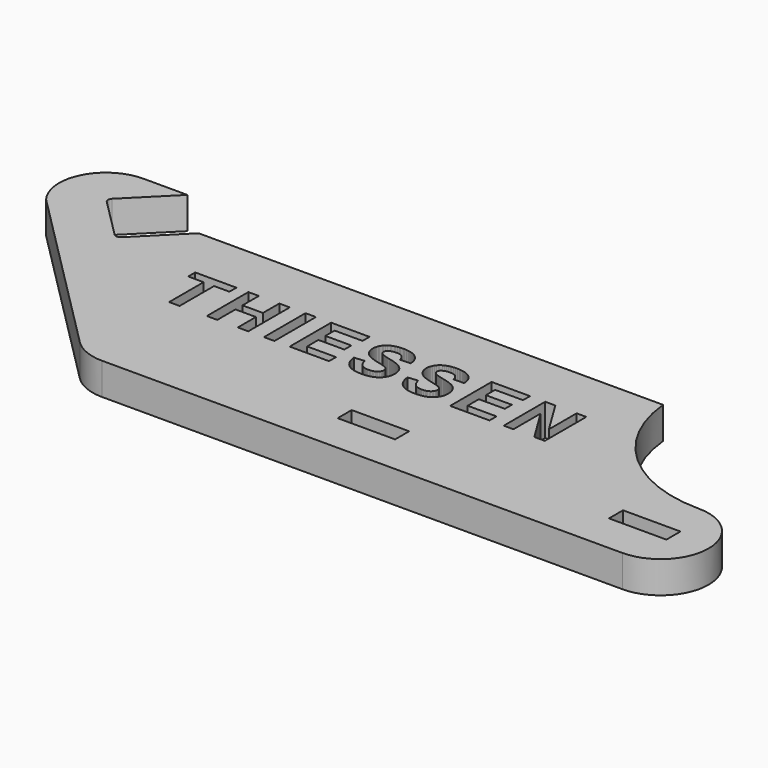
from build123d import *

# Parameters (mm, degrees)
F0_W     = 45.72
F0_H     = 13.97
F0_W_2   = 8.33755
F0_H_2   = 41.275
F1_DEPTH = 25.4


# Not quite as in the source:
# - ends of sketch curves that miss each other by under 0.0002 mm in the source are joined


with BuildPart() as f1:
    # F0 (on Top) → F1 (new body)
    with BuildSketch(Plane.XY):
        with BuildLine():
            Line((-272.2032402, 70.4585586), (-238.976281, 103.6855178))
            Line((-238.976281, 103.6855178), (-273.9992996, 103.6855178))
            ThreePointArc((-273.9992996, 103.6855178), (-307.3025453403, 83.0573981079), (-303.6687029451, 44.0520184737))
            Line((-303.6687029451, 44.0520184737), (-167.3257004, -92.790645))
            ThreePointArc((-167.3257004, -92.790645), (-155.2579794367, -100.8540315519), (-141.0231368, -103.6855178))
            Line((-141.0231368, -103.6855178), (273.096736, -103.6855178))
            ThreePointArc((273.096736, -103.6855178), (311.196736, -65.5855178), (273.096736, -27.4855178))
            ThreePointArc((273.096736, -27.4855178), (202.2970835909, -0.11388545), (168.321736, 67.7644822))
            Line((168.321736, 67.7644822), (-201.2592114, 67.7644822))
            Line((-201.2592114, 67.7644822), (-235.3841876, 33.639506))
            ThreePointArc((-235.3841876, 33.639506), (-238.078264, 32.5235824), (-240.7723408363, 33.6395055637))
            Line((-240.7723408363, 33.6395055637), (-272.2032402, 65.0704058))
            ThreePointArc((-272.2032402, 65.0704058), (-273.3191638, 67.7644822), (-272.2032402, 70.4585586))
        make_face()
        with Locations((44.496736, -65.5855178)):
            Rectangle(F0_W, F0_H, mode=Mode.SUBTRACT)
        with Locations((260.396736, -65.5855178)):
            Rectangle(F0_W, F0_H, mode=Mode.SUBTRACT)
        Polygon((-149.3758506, -16.014827), (-157.7134006, -16.014827), (-157.7134006, 18.284698), (-169.9720756, 18.284698), (-169.9720756, 25.260173), (-137.1584506, 25.260173), (-137.1584506, 18.284698), (-149.3758506, 18.284698), align=None, mode=Mode.SUBTRACT)
        Polygon((-119.3595276, -16.014827), (-127.6970776, -16.014827), (-127.6970776, 25.260173), (-119.3595276, 25.260173), (-119.3595276, 8.997823), (-103.0559026, 8.997823), (-103.0559026, 25.260173), (-94.7183526, 25.260173), (-94.7183526, -16.014827), (-103.0559026, -16.014827), (-103.0559026, 2.022348), (-119.3595276, 2.022348), align=None, mode=Mode.SUBTRACT)
        with Locations((-78.075155, 4.622673)):
            Rectangle(F0_W_2, F0_H_2, mode=Mode.SUBTRACT)
        Polygon((-30.4757074, -16.014827), (-61.8034324, -16.014827), (-61.8034324, 25.260173), (-31.2599324, 25.260173), (-31.2599324, 18.284698), (-53.4658824, 18.284698), (-53.4658824, 9.121648), (-32.7871074, 9.121648), (-32.7871074, 2.146173), (-53.4658824, 2.146173), (-53.4658824, -9.039352), (-30.4757074, -9.039352), align=None, mode=Mode.SUBTRACT)
        Polygon((-21.2402166, -3.6873688), (-21.3858094, -2.641727), (-13.2959094, -1.857502), (-13.0892042, -2.8459176), (-12.8354074, -3.7664898), (-12.5344936, -4.6191678), (-12.1864882, -5.4040024), (-11.7913912, -6.1209682), (-11.3491772, -6.7700398), (-10.8598716, -7.351268), (-10.3234744, -7.8646274), (-9.7390966, -8.3140804), (-9.1058492, -8.7036148), (-8.423783, -9.0332052), (-7.6928472, -9.302877), (-6.9130418, -9.5126302), (-6.0843922, -9.6624394), (-5.2068984, -9.75233), (-4.2805604, -9.782302), (-3.3043876, -9.755632), (-2.3902924, -9.6756728), (-1.5382748, -9.5424244), (-0.7483094, -9.355836), (-0.020447, -9.1159584), (0.6453632, -8.8227662), (1.2490958, -8.4762848), (1.7907508, -8.0764888), (2.4148288, -7.4918316), (2.925445, -6.8750688), (3.3225994, -6.2262004), (3.6062666, -5.5452264), (3.776472, -4.8321722), (3.8332156, -4.086987), (3.7377878, -3.158236), (3.4515552, -2.3264876), (2.9744924, -1.5917926), (2.46507, -1.0939018), (1.7955006, -0.6295644), (0.9657842, -0.198755), (-0.0240792, 0.1985264), (-0.448564, 0.337566), (-0.9900412, 0.501269), (-1.6485108, 0.68961), (-2.4239982, 0.9026144), (-3.3164526, 1.1402568), (-4.3258994, 1.4025372), (-5.4523386, 1.689481), (-6.6957956, 2.0010628), (-7.7848206, 2.2833584), (-8.8183212, 2.576195), (-9.7962974, 2.8796234), (-10.7187492, 3.1935928), (-11.5856512, 3.518154), (-12.3970542, 3.8532816), (-13.1529328, 4.1989756), (-13.853287, 4.555236), (-14.4980914, 4.9220882), (-15.0873968, 5.2994814), (-15.6211524, 5.6874664), (-16.0993836, 6.0860178), (-16.7589962, 6.718173), (-17.3557692, 7.375017), (-17.889728, 8.0565498), (-18.3608726, 8.762746), (-18.7691776, 9.493631), (-19.1146938, 10.2491794), (-19.3973704, 11.0294166), (-19.6172328, 11.8343172), (-19.774281, 12.6639066), (-19.868515, 13.5181594), (-19.8999094, 14.3971264), (-19.863435, 15.2903682), (-19.7540372, 16.166973), (-19.5716906, 17.0268646), (-19.3163952, 17.8701192), (-18.988151, 18.6966606), (-18.586958, 19.506565), (-18.1128416, 20.2997562), (-17.641443, 20.966049), (-17.1207938, 21.591397), (-16.5508686, 22.1758002), (-15.9317182, 22.7192586), (-15.2632918, 23.2217976), (-14.5456148, 23.6833664), (-13.7786872, 24.1039904), (-12.9624836, 24.483695), (-12.1978928, 24.7852692), (-11.3989104, 25.0513596), (-10.5655364, 25.2819662), (-9.6977454, 25.477089), (-8.7955882, 25.6367534), (-7.859014, 25.760934), (-6.8880482, 25.8496308), (-5.8826908, 25.9028438), (-4.8429164, 25.920573), (-3.7529008, 25.9031994), (-2.702052, 25.8510278), (-1.6903954, 25.7640582), (-0.7179564, 25.6423414), (0.2152904, 25.4858266), (1.1093704, 25.2945392), (1.9642328, 25.0684792), (2.779903, 24.8076212), (3.5563556, 24.5119906), (4.2936414, 24.1815874), (4.991735, 23.8164116), (5.650611, 23.4164378), (6.2702948, 22.9816914), (6.8507864, 22.5121724), (7.479284, 21.9282518), (8.0559656, 21.3126574), (8.5808312, 20.6653892), (9.0539316, 19.9864472), (9.4751906, 19.275806), (9.8446844, 18.533491), (10.1623622, 17.7594768), (10.4282494, 16.9537888), (10.6423206, 16.116427), (10.8046266, 15.2473914), (10.9150912, 14.3466566), (10.9737906, 13.414248), (2.6362406, 13.042773), (2.424049, 14.0562584), (2.1439124, 14.9701504), (1.7958054, 15.7844998), (1.3797788, 16.4992812), (0.8957818, 17.1144692), (0.3438652, 17.6301146), (-0.1942338, 18.0008784), (-0.8041132, 18.3146192), (-1.4857476, 18.5713116), (-2.239137, 18.7709556), (-3.0643322, 18.9135766), (-3.9612824, 18.9991238), (-4.9299876, 19.027648), (-5.9345068, 18.9971426), (-6.874764, 18.9055756), (-7.7507338, 18.752947), (-8.5623908, 18.5393076), (-9.3098112, 18.2646066), (-9.9929188, 17.9288694), (-10.6117644, 17.5320706), (-11.1901732, 17.0119802), (-11.6033296, 16.4107114), (-11.8512082, 15.7282642), (-11.9338344, 14.9646386), (-11.8564152, 14.2574772), (-11.6241322, 13.603224), (-11.23696, 13.0018282), (-10.6949494, 12.4533152), (-10.3345234, 12.1870216), (-9.8839782, 11.9185182), (-9.3433392, 11.6477796), (-8.7125556, 11.3748566), (-7.9916782, 11.0996984), (-7.1806816, 10.8223558), (-6.2795658, 10.542778), (-5.2883308, 10.2609904), (-4.207002, 9.976993), (-3.0355286, 9.6907858), (-1.9558, 9.4287848), (-0.9284208, 9.1651836), (0.0465836, 8.8999568), (0.9692386, 8.6331044), (1.8394934, 8.3646518), (2.6573988, 8.0945736), (3.4229548, 7.8228698), (4.136136, 7.5495658), (4.7969424, 7.2746616), (5.405374, 6.9981064), (5.9614562, 6.7199764), (6.7682872, 6.2586362), (7.5234038, 5.7513474), (8.226806, 5.19811), (8.8784938, 4.598924), (9.4784672, 3.9538148), (10.0267516, 3.2627316), (10.5232962, 2.5257252), (10.909427, 1.8411444), (11.244072, 1.1174222), (11.5272312, 0.3545586), (11.7589046, -0.4474464), (11.9390922, -1.2886182), (12.067794, -2.1689314), (12.14501, -3.088386), (12.1707656, -4.0470074), (12.1399554, -4.9267364), (12.047601, -5.7923938), (11.8936516, -6.6439542), (11.6781072, -7.4814684), (11.4010186, -8.3048856), (11.0623096, -9.1142058), (10.6620564, -9.9094798), (10.2002082, -10.6906568), (9.6820482, -11.4399568), (9.1128596, -12.139549), (8.4926424, -12.7894334), (7.8213966, -13.3895846), (7.0991222, -13.9400534), (6.3258192, -14.440789), (5.5014876, -14.8918168), (4.6261274, -15.2931622), (3.8876986, -15.5792678), (3.1138114, -15.8352744), (2.3044404, -16.0611566), (1.459611, -16.2569144), (0.5793232, -16.4225732), (-0.336423, -16.5581076), (-1.2876276, -16.6635176), (-2.274316, -16.7388032), (-3.2964628, -16.7839898), (-4.354068, -16.799052), (-5.4535578, -16.7805862), (-6.515989, -16.7252396), (-7.541387, -16.6329614), (-8.529701, -16.5038024), (-9.4809564, -16.3377372), (-10.3951532, -16.1347404), (-11.2723168, -15.8948628), (-12.1123964, -15.618079), (-12.9154428, -15.304389), (-13.6814306, -14.9537928), (-14.4103344, -14.566265), (-15.102205, -14.1418564), (-15.757017, -13.6805416), (-16.3747704, -13.1823206), (-17.000093, -12.6063248), (-17.5854614, -11.991213), (-18.1308248, -11.3369598), (-18.636234, -10.6435398), (-19.1016382, -9.9110038), (-19.5270882, -9.1393264), (-19.9125586, -8.3285076), (-20.2580494, -7.4785474), (-20.5635606, -6.5894712), (-20.8290922, -5.6612282), (-21.0546442, -4.6938692), align=None, mode=Mode.SUBTRACT)
        Polygon((21.323681, -3.6873688), (21.1780882, -2.641727), (29.2679882, -1.857502), (29.4746934, -2.8459176), (29.7284902, -3.7664898), (30.029404, -4.6191678), (30.3774094, -5.4040024), (30.7725318, -6.1209682), (31.2147204, -6.7700398), (31.704026, -7.351268), (32.2404232, -7.8646274), (32.824801, -8.3140804), (33.4580484, -8.7036148), (34.14014, -9.0332052), (34.8710758, -9.302877), (35.6508558, -9.5126302), (36.4795054, -9.6624394), (37.3569992, -9.75233), (38.2833626, -9.782302), (39.25951, -9.755632), (40.1736052, -9.6756728), (41.0256482, -9.5424244), (41.8155882, -9.355836), (42.5434506, -9.1159584), (43.2092608, -8.8227662), (43.8129934, -8.4762848), (44.3546484, -8.0764888), (44.9787264, -7.4918316), (45.4893426, -6.8750688), (45.886497, -6.2262004), (46.1701642, -5.5452264), (46.3403696, -4.8321722), (46.3971132, -4.086987), (46.3017108, -3.158236), (46.0154528, -2.3264876), (45.53839, -1.5917926), (45.0289676, -1.0939018), (44.3593982, -0.6295644), (43.5296818, -0.198755), (42.5398438, 0.1985264), (42.1153336, 0.337566), (41.5738564, 0.501269), (40.9153868, 0.68961), (40.1399248, 0.9026144), (39.2474704, 1.1402568), (38.2379982, 1.4025372), (37.111559, 1.689481), (35.8681274, 2.0010628), (34.7791024, 2.2833584), (33.7456018, 2.576195), (32.7676256, 2.8796234), (31.8451738, 3.1935928), (30.9782464, 3.518154), (30.1668434, 3.8532816), (29.4109648, 4.1989756), (28.710636, 4.555236), (28.0658062, 4.9220882), (27.4765262, 5.2994814), (26.9427452, 5.6874664), (26.464514, 6.0860178), (25.8049268, 6.718173), (25.2081284, 7.375017), (24.6741696, 8.0565498), (24.2030504, 8.762746), (23.79472, 9.493631), (23.4492292, 10.2491794), (23.1665272, 11.0294166), (22.9466648, 11.8343172), (22.7896166, 12.6639066), (22.695408, 13.5181594), (22.6639882, 14.3971264), (22.7004626, 15.2903682), (22.8098604, 16.166973), (22.9922324, 17.0268646), (23.2475278, 17.8701192), (23.575772, 18.6966606), (23.9769396, 19.506565), (24.451056, 20.2997562), (24.9224546, 20.966049), (25.4431292, 21.591397), (26.013029, 22.1758002), (26.6321794, 22.7192586), (27.3006058, 23.2217976), (28.0182828, 23.6833664), (28.7852104, 24.1039904), (29.601414, 24.483695), (30.3660048, 24.7852692), (31.1649872, 25.0513596), (31.9983612, 25.2819662), (32.8661522, 25.477089), (33.7683348, 25.6367534), (34.7048836, 25.760934), (35.6758494, 25.8496308), (36.6812322, 25.9028438), (37.7209812, 25.920573), (38.8110222, 25.9031994), (39.8618456, 25.8510278), (40.8735022, 25.7640582), (41.8459412, 25.6423414), (42.7792134, 25.4858266), (43.673268, 25.2945392), (44.5281304, 25.0684792), (45.3438006, 24.8076212), (46.1202786, 24.5119906), (46.857539, 24.1815874), (47.5556326, 23.8164116), (48.2145086, 23.4164378), (48.8342178, 22.9816914), (49.4147094, 22.5121724), (50.0431816, 21.9282518), (50.6198632, 21.3126574), (51.1447542, 20.6653892), (51.6178292, 19.9864472), (52.0391136, 19.275806), (52.408582, 18.533491), (52.7262598, 17.7594768), (52.992147, 16.9537888), (53.2062436, 16.116427), (53.3685242, 15.2473914), (53.4790142, 14.3466566), (53.5376882, 13.414248), (45.2001382, 13.042773), (44.9879466, 14.0562584), (44.70781, 14.9701504), (44.3597284, 15.7844998), (43.9436764, 16.4992812), (43.4597048, 17.1144692), (42.9077628, 17.6301146), (42.3696638, 18.0008784), (41.7598098, 18.3146192), (41.0781754, 18.5713116), (40.3247606, 18.7709556), (39.4995908, 18.9135766), (38.6026406, 18.9991238), (37.63391, 19.027648), (36.6293908, 18.9971426), (35.6891336, 18.9055756), (34.8131892, 18.752947), (34.0015068, 18.5393076), (33.2541118, 18.2646066), (32.5709788, 17.9288694), (31.9521586, 17.5320706), (31.3737498, 17.0119802), (30.9605934, 16.4107114), (30.7126894, 15.7282642), (30.6300632, 14.9646386), (30.7074824, 14.2574772), (30.9397908, 13.603224), (31.3269376, 13.0018282), (31.8689482, 12.4533152), (32.2293742, 12.1870216), (32.6799194, 11.9185182), (33.2205838, 11.6477796), (33.851342, 11.3748566), (34.5722194, 11.0996984), (35.383216, 10.8223558), (36.2843318, 10.542778), (37.2755668, 10.2609904), (38.356921, 9.976993), (39.528369, 9.6907858), (40.608123, 9.4287848), (41.6354768, 9.1651836), (42.6104812, 8.8999568), (43.5331362, 8.6331044), (44.4034164, 8.3646518), (45.2213218, 8.0945736), (45.9868524, 7.8228698), (46.7000336, 7.5495658), (47.36084, 7.2746616), (47.9692716, 6.9981064), (48.5253538, 6.7199764), (49.3321848, 6.2586362), (50.0873014, 5.7513474), (50.7907036, 5.19811), (51.4423914, 4.598924), (52.0423902, 3.9538148), (52.5906492, 3.2627316), (53.0872192, 2.5257252), (53.4733246, 1.8411444), (53.8079696, 1.1174222), (54.0911288, 0.3545586), (54.3228022, -0.4474464), (54.5029898, -1.2886182), (54.6316916, -2.1689314), (54.708933, -3.088386), (54.7346632, -4.0470074), (54.7038784, -4.9267364), (54.6114986, -5.7923938), (54.4575492, -6.6439542), (54.2420302, -7.4814684), (53.9649162, -8.3048856), (53.6262326, -9.1142058), (53.225954, -9.9094798), (52.7641058, -10.6906568), (52.2459458, -11.4399568), (51.6767572, -12.139549), (51.05654, -12.7894334), (50.3853196, -13.3895846), (49.6630452, -13.9400534), (48.8897422, -14.440789), (48.0654106, -14.8918168), (47.1900504, -15.2931622), (46.4516216, -15.5792678), (45.677709, -15.8352744), (44.8683634, -16.0611566), (44.023534, -16.2569144), (43.1432462, -16.4225732), (42.2274746, -16.5581076), (41.27627, -16.6635176), (40.2895816, -16.7388032), (39.2674348, -16.7839898), (38.2098296, -16.799052), (37.1103398, -16.7805862), (36.0479086, -16.7252396), (35.022536, -16.6329614), (34.034222, -16.5038024), (33.0829412, -16.3377372), (32.1687444, -16.1347404), (31.2915808, -15.8948628), (30.4515012, -15.618079), (29.6484548, -15.304389), (28.8824924, -14.9537928), (28.1535632, -14.566265), (27.4616926, -14.1418564), (26.8068806, -13.6805416), (26.1891272, -13.1823206), (25.5638046, -12.6063248), (24.9784362, -11.991213), (24.4330728, -11.3369598), (23.9276636, -10.6435398), (23.4622594, -9.9110038), (23.0368094, -9.1393264), (22.651339, -8.3285076), (22.3058736, -7.4785474), (22.0003624, -6.5894712), (21.7348308, -5.6612282), (21.5092534, -4.6938692), align=None, mode=Mode.SUBTRACT)
        Polygon((97.2160108, -16.014827), (65.8882858, -16.014827), (65.8882858, 25.260173), (96.4317858, 25.260173), (96.4317858, 18.284698), (74.2258358, 18.284698), (74.2258358, 9.121648), (94.9046108, 9.121648), (94.9046108, 2.146173), (74.2258358, 2.146173), (74.2258358, -9.039352), (97.2160108, -9.039352), align=None, mode=Mode.SUBTRACT)
        Polygon((116.2531838, -16.014827), (108.5347588, -16.014827), (108.5347588, 25.260173), (116.6188422, 25.260173), (133.5061338, -2.3469854), (133.5061338, 25.260173), (141.2245588, 25.260173), (141.2245588, -16.014827), (132.8870088, -16.014827), (116.2531838, 11.0222284), align=None, mode=Mode.SUBTRACT)
    extrude(amount=F1_DEPTH)


solid = f1.part
